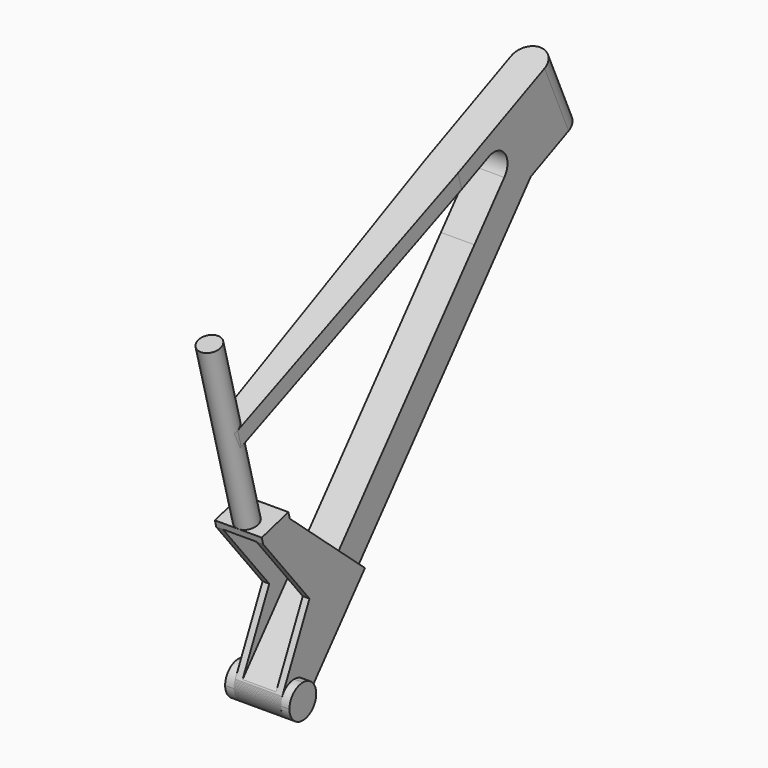
from build123d import *
from build123d import SkipClean  # not in build123d's __all__

# Parameters (mm, degrees)
F5_DEPTH  = 48
F7_W      = 50
F7_H      = 50
F8_REACH  = 912.7734613462
F10_R     = 16.5
F11_DEPTH = 280
F4_W      = 50
F4_H      = 25
F12_DEPTH = 621
F14_DEPTH = 50
F16_DEPTH = 50
F19_DEPTH = 35
F20_W     = 50
F20_H     = 250
F21_REACH = 742.8364387972
F24_DEPTH = 142
F25_DEPTH = 270
F22_W     = 10
F22_H     = 51.5
F26_DEPTH = 10


# Not quite as in the source:
# - an extrude ends at something that could not be found from the text; its depth is read off the source's solid


with BuildPart() as f2:
    # F1 (on Right) → F2 (revolve)
    with BuildSketch(Plane.YZ):
        Polygon((502.8386364411, 639.7222130194), (480, 629.5537969425), (524.7410307383, 529.0637966018), (547.5796671794, 539.2322126787), align=None)
    revolve(axis=Axis((0, 502.3705153692, 579.3087967721), (0, 0.4067366431, -0.9135454576)))

    f8_end = f2.faces().sort_by_distance((0, 479.5318789281, 569.1403806952))[0]
    # F7 (on line) → F8 (join, up to a face of the model that its end follows)
    with BuildSketch(Plane(origin=(0, 0, 0), x_dir=(1, 0, 0), z_dir=(0, 0.6462360214, 0.7631376053))):
        Rectangle(F7_W, F7_H)
    f8_long = extrude(amount=F8_REACH, mode=Mode.PRIVATE)
    add(split(f8_long, bisect_by=f8_end, keep=Keep.ALL, mode=Mode.PRIVATE).solids().sort_by_distance((0, 0, 0))[0])



with BuildPart() as f5:
    # F0 (on Right) → F5 (new body, symmetric)
    with BuildSketch(Plane.YZ):
        with BuildLine():
            Line((0, 0), (0, 25))
            ThreePointArc((0, 25), (-17.6776695297, 17.6776695297), (-25, 0))
            Line((-25, 0), (0, 0))
        make_face()
        with BuildLine():
            Line((15, 17.7134416851), (14.2405756119, 20.5476520858))
            ThreePointArc((14.2405756119, 20.5476520858), (7.4601842422, 23.8609650072), (0, 25))
            Line((0, 25), (0, 0))
            Line((0, 0), (15, 17.7134416851))
        make_face()
        with BuildLine():
            ThreePointArc((16.1559005349, 19.078440133), (15.2159812854, 19.8361768878), (14.2405756119, 20.5476520858))
            Line((14.2405756119, 20.5476520858), (15, 17.7134416851))
            Line((15, 17.7134416851), (16.1559005349, 19.078440133))
        make_face()
        with BuildLine():
            Line((16.1559005349, 19.078440133), (15, 17.7134416851))
            Line((15, 17.7134416851), (0, 0))
            Line((0, 0), (25, 0))
            ThreePointArc((25, 0), (22.6814628427, 10.5143351342), (16.1559005349, 19.078440133))
        make_face()
        with BuildLine():
            Line((0, 0), (-25, 0))
            ThreePointArc((-25, 0), (0, -25), (25, 0))
            Line((25, 0), (0, 0))
        make_face()
    extrude(amount=F5_DEPTH, both=True)


with BuildPart() as f11:
    # F10 (on line) → F11 (new body)
    with BuildSketch(Plane(origin=(0, -132.8330735009, 495.739779231), x_dir=(1, 0, 0), z_dir=(0, -0.2588190451, 0.9659258263))):
        with Locations((0, 19.0734634568)):
            Circle(F10_R)
    extrude(amount=-F11_DEPTH)


with BuildPart() as f2_1:
    add(f2.part, clean=False)

    add(f11.part)  # F12 merges F11
    # F4 (on line) → F12 (join)
    with BuildSketch(Plane(origin=(0, 634.5161688048, 282.504799644), x_dir=(1, 0, 0), z_dir=(0, -0.9135454576, -0.4067366431))):
        with Locations((0, 367.3924228621)):
            Rectangle(F4_W, F4_H)
    extrude(amount=F12_DEPTH)

    # F13 (on face) → F14 (join, through all)
    with BuildSketch(Plane.YZ.offset(25)):
        Polygon((509.5918311512, 563.0894559697), (480, 629.5537969425), (349.0007462707, 571.2291714281), (349.0007462707, 450.8191807925), (454.1720638958, 497.6444682709), align=None)
        Polygon((524.7410307383, 529.0637966018), (509.5918311512, 563.0894559697), (454.1720638958, 497.6444682709), align=None)
    extrude(amount=-F14_DEPTH)

    # F15 (on face) → F16 (cut, through all)
    with BuildSketch(Plane.YZ.offset(25)):
        with BuildLine():
            Line((375.5236657091, 555.6720290176), (349.0007462707, 543.8632644655))
            Line((349.0007462707, 543.8632644655), (349.0007462707, 450.8191807925))
            Line((349.0007462707, 450.8191807925), (404.770521919, 516.6774920417))
            ThreePointArc((404.770521919, 516.6774920417), (405.6918470512, 547.8337055512), (375.5236657091, 555.6720290176))
        make_face()
    extrude(amount=-F16_DEPTH, mode=Mode.SUBTRACT)

    # F18 (on Right) → F19 (join, symmetric)
    with BuildSketch(Plane.YZ):
        with BuildLine():
            ThreePointArc((19.078440133, -16.1559005349), (23.4729738564, -8.6034585103), (25, 0))
            ThreePointArc((25, 0), (5.8117636963, 24.3150859085), (-22.2978722191, 11.3050826844))
            ThreePointArc((-22.2978722191, 11.3050826844), (-13.8245284036, -20.8298443206), (19.078440133, -16.1559005349))
        make_face()
        with BuildLine():
            ThreePointArc((-22.2978722191, 11.3050826844), (5.8117636963, 24.3150859085), (25, 0))
            ThreePointArc((25, 0), (23.4729738564, -8.6034585103), (19.078440133, -16.1559005349))
            Line((19.078440133, -16.1559005349), (132.169743877, 117.393180396))
            Line((132.169743877, 117.393180396), (58.1101733819, 181.729680453))
            Line((58.1101733819, 181.729680453), (28.6130073485, 119.2105305473))
            Line((28.6130073485, 119.2105305473), (-22.2978722191, 11.3050826844))
        make_face()
        Polygon((-57.8779660563, 225.9466092245), (28.6130073485, 119.2105305473), (58.1101733819, 181.729680453), (-8.1327860024, 239.2757900473), align=None)
    extrude(amount=F19_DEPTH, both=True)

    f21_end = Plane(origin=(0, -30.2261892372, 233.3558804925), x_dir=(0, 0.9659258263, 0.2588190451), z_dir=(0, -0.2588190451, 0.9659258263))
    # F20 (on face) → F21 (cut, up to a plane its end follows)
    with BuildSketch(Plane(origin=(0, -19.078440133, 16.1559005349), x_dir=(1, 0, 0), z_dir=(0, -0.7631376053, 0.6462360214))):
        with Locations((0, 100)):
            Rectangle(F20_W, F20_H)
    f21_long = extrude(amount=F21_REACH, mode=Mode.PRIVATE)
    add(split(f21_long, bisect_by=f21_end, keep=Keep.BOTTOM, mode=Mode.PRIVATE), mode=Mode.SUBTRACT)

    # F23 (on face) → F24 (cut)
    with BuildSketch(Plane(origin=(0, -132.8330735009, 495.739779231), x_dir=(1, 0, 0), z_dir=(0, -0.2588190451, 0.9659258263))):
        with BuildLine():
            ThreePointArc((0, 2.5734634568), (-11.5522090109, 7.2922722195), (-16.4968222509, 18.7496492786))
            Line((-16.4968222509, 18.7496492786), (-18.4926110681, 120.4257820466))
            Line((-18.4926110681, 120.4257820466), (-58.093066782, 121.2030947208))
            Line((-58.093066782, 121.2030947208), (-58.093066782, 2.5734634568))
            Line((-58.093066782, 2.5734634568), (0, 2.5734634568))
        make_face()
        Polygon((-58.093066782, 121.2030947208), (-18.4926110681, 120.4257820466), (-25, 451.9469005739), (-58.093066782, 452.5964804784), align=None)
        with BuildLine():
            Line((18.4783664089, 119.7000830905), (16.4968222509, 18.7496492786))
            ThreePointArc((16.4968222509, 18.7496492786), (11.5522090109, 7.2922722195), (0, 2.5734634568))
            Line((0, 2.5734634568), (64.5229642251, 2.5734634568))
            Line((64.5229642251, 2.5734634568), (64.5229642251, 118.796279111))
            Line((64.5229642251, 118.796279111), (18.4783664089, 119.7000830905))
        make_face()
        Polygon((25, 451.9469005739), (18.4783664089, 119.7000830905), (64.5229642251, 118.796279111), (64.5229642251, 451.171108971), align=None)
    with SkipClean():  # cleaning this boolean's faces spoils the solid; the shape is the same uncleaned
        extrude(amount=-F24_DEPTH, mode=Mode.SUBTRACT)

    # F23 (on face) → F25 (cut, through all)
    with BuildSketch(Plane(origin=(0, -132.8330735009, 495.739779231), x_dir=(1, 0, 0), z_dir=(0, -0.2588190451, 0.9659258263))):
        with BuildLine():
            Line((18.4783664089, 119.7000830905), (16.4968222509, 18.7496492786))
            ThreePointArc((16.4968222509, 18.7496492786), (11.5522090109, 7.2922722195), (0, 2.5734634568))
            Line((0, 2.5734634568), (64.5229642251, 2.5734634568))
            Line((64.5229642251, 2.5734634568), (64.5229642251, 118.796279111))
            Line((64.5229642251, 118.796279111), (18.4783664089, 119.7000830905))
        make_face()
        with BuildLine():
            ThreePointArc((0, 2.5734634568), (-11.5522090109, 7.2922722195), (-16.4968222509, 18.7496492786))
            Line((-16.4968222509, 18.7496492786), (-18.4926110681, 120.4257820466))
            Line((-18.4926110681, 120.4257820466), (-58.093066782, 121.2030947208))
            Line((-58.093066782, 121.2030947208), (-58.093066782, 2.5734634568))
            Line((-58.093066782, 2.5734634568), (0, 2.5734634568))
        make_face()
    extrude(amount=-F25_DEPTH, mode=Mode.SUBTRACT)

    # F22 (on face) → F26 (join)
    with BuildSketch(Plane(origin=(0, -60.3637408722, 225.28054787), x_dir=(1, 0, 0), z_dir=(0, -0.2588190451, 0.9659258263))):
        Polygon((-25, 54.0734634568), (-25, 2.5734634568), (0, 2.5734634568), (35, 2.5734634568), (35, 54.0734634568), align=None)
        with BuildLine():
            ThreePointArc((16.5, 19.0734634568), (11.6672618896, 7.4062015672), (0, 2.5734634568))
            ThreePointArc((0, 2.5734634568), (-11.6672618896, 30.7407253463), (16.5, 19.0734634568))
        make_face(mode=Mode.SUBTRACT)
        with Locations((-30, 28.3234634568)):
            Rectangle(F22_W, F22_H)
    extrude(amount=F26_DEPTH)


solid = Compound([f5.part, f2_1.part])
